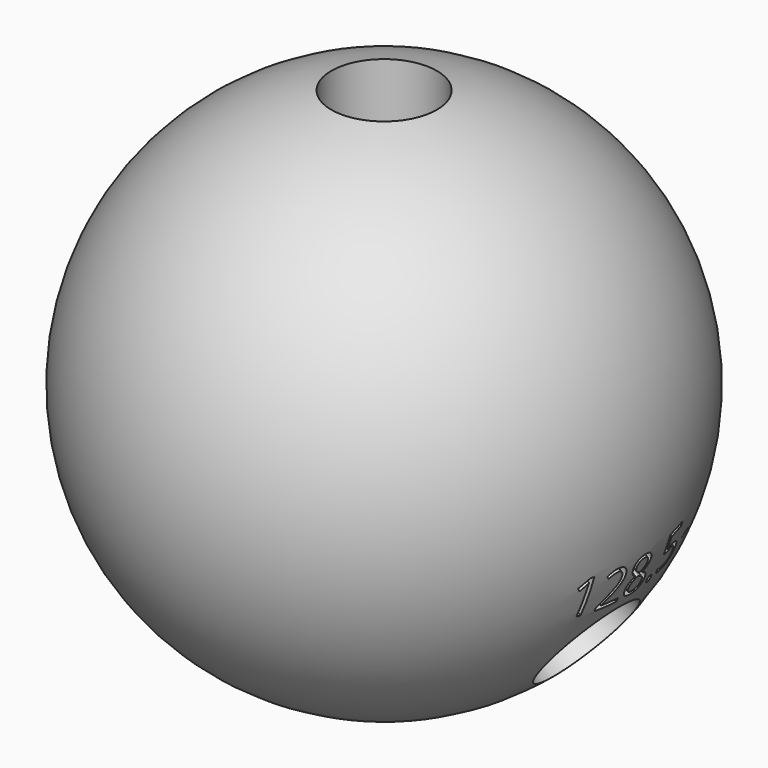
from build123d import *

# Parameters (mm, degrees)
F4_R          = 3.175
F5_DEPTH      = 50.8
F7_ANGLE      = 128.5
F8_ANGLE      = -128.6
F10_TEXT_SIZE = 3.259410409
F11_DEPTH     = 6.35
F13_TEXT_SIZE = 3.7313827003
F14_DEPTH     = 6.35


# Not quite as in the source:
# - Text() gives the source's letters only with a copy of the font that has no kerning and outlines rounded to 1/6400 em; it was checked with that copy


with BuildPart() as f2:
    # F0 (on Front) → F2 (revolve)
    with BuildSketch(Plane.XZ):
        with BuildLine():
            Line((0, -15.875), (0, 15.875))
            ThreePointArc((0, 15.875), (-15.875, 0), (0, -15.875))
        make_face()
    revolve(axis=Axis((0, 0, 0), (0, 0, 1)))

    # F10 (on offset) → F11 (cut)
    with BuildSketch(Plane(origin=(14.908685388, 0, -11.8589038279), x_dir=(0, 1, 0), z_dir=(0.7826081569, 0, -0.6225146366))):
        with Locations((-4.1261431761, 3.8076173514)):
            Text('128.5', F10_TEXT_SIZE, font='Open Sans', text_align=(TextAlign.LEFT, TextAlign.BOTTOM))
    extrude(amount=-F11_DEPTH, mode=Mode.SUBTRACT)

    # F13 (on offset) → F14 (cut)
    with BuildSketch(Plane(origin=(-14.8879649996, 0, -11.8849063173), x_dir=(0, -1, 0), z_dir=(-0.7815204724, 0, -0.6238795967))):
        with Locations((-4.5592235401, 3.5901465453)):
            Text('128.6', F13_TEXT_SIZE, font='Open Sans', text_align=(TextAlign.LEFT, TextAlign.BOTTOM))
    extrude(amount=-F14_DEPTH, mode=Mode.SUBTRACT)


with BuildPart() as f5:
    # F4 (on offset) → F5 (new body)
    with BuildSketch(Plane.XY.offset(6.35)):
        Circle(F4_R)
    extrude(amount=F5_DEPTH)


with BuildPart() as f7_1:
    # F7: copy of F5
    add(f5.part.rotate(Axis((0, 22.3991125822, 0), (0, 1, 0)), F7_ANGLE))


with BuildPart() as f8_1:
    # F8: copy of F5
    add(f5.part.rotate(Axis((0, 22.3991125822, 0), (0, 1, 0)), F8_ANGLE))


with BuildPart() as f2_1:
    add(f2.part)

    # F15: cut F5, F7_1, F8_1
    add(f5.part, mode=Mode.SUBTRACT)
    add(f7_1.part, mode=Mode.SUBTRACT)
    add(f8_1.part, mode=Mode.SUBTRACT)


solid = f2_1.part
